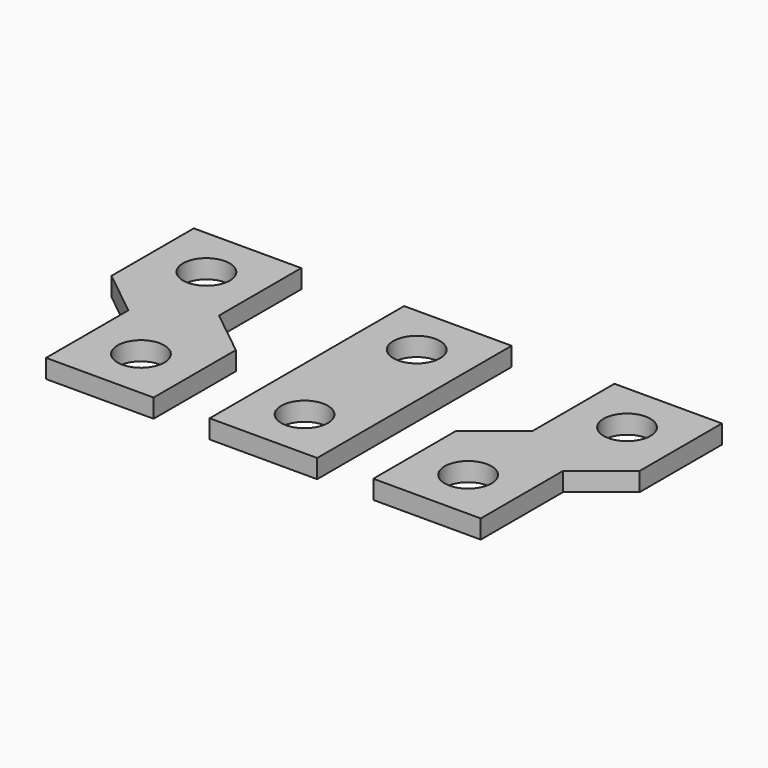
from build123d import *

# Parameters (mm, degrees)
F0_R     = 5
F1_DEPTH = 4
F0_W     = 23
F0_H     = 52


# Not quite as in the source:
# - a feature names something its author has since deleted; it is built from what else it names


with BuildPart() as f1:
    # F0 (on Top) → F1 (new body)
    with BuildSketch(Plane.XY):
        Polygon((-46.5, -26), (-23.5, -26), (-23.5, -4), (-33.5, 4), (-33.5, 26), (-56.5, 26), (-56.5, 4), (-46.5, -4), align=None)
        with Locations((-35, -15)):
            Circle(F0_R, mode=Mode.SUBTRACT)
        with Locations((-45, 15)):
            Circle(F0_R, mode=Mode.SUBTRACT)
    extrude(amount=F1_DEPTH)


with BuildPart() as f1b:
    # F0 (on Top) → F1, piece 2 (new body)
    with BuildSketch(Plane.XY):
        Rectangle(F0_W, F0_H)
        with Locations((0, -15)):
            Circle(F0_R, mode=Mode.SUBTRACT)
        with Locations((0, 15)):
            Circle(F0_R, mode=Mode.SUBTRACT)
    extrude(amount=F1_DEPTH)


with BuildPart() as f1c:
    # F0 (on Top) → F1, piece 3 (new body)
    with BuildSketch(Plane.XY):
        Polygon((56.5, 4), (56.5, 26), (33.5, 26), (33.5, 4), (23.5, -4), (23.5, -26), (46.5, -26), (46.5, -4), align=None)
        with Locations((35, -15)):
            Circle(F0_R, mode=Mode.SUBTRACT)
        with Locations((45, 15)):
            Circle(F0_R, mode=Mode.SUBTRACT)
    extrude(amount=F1_DEPTH)


solid = Compound([f1.part, f1b.part, f1c.part])
